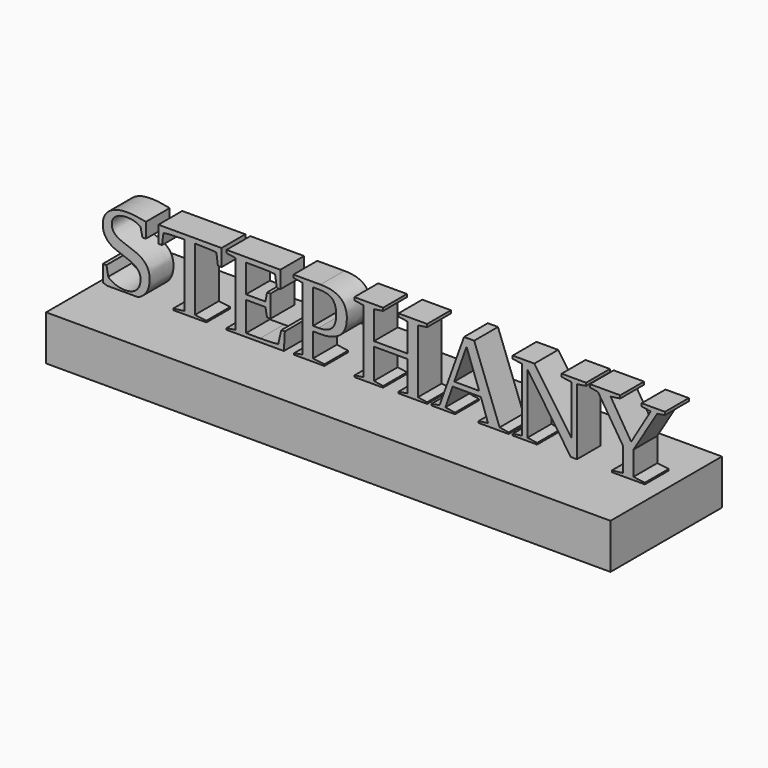
from build123d import *

# Parameters (mm, degrees)
F0_TEXT_SIZE  = 46.7684339835
F1_DEPTH      = 12.7
F2_W          = 240.8891022205
F2_H          = 19.2134454846
F3_DEPTH      = 40.386
F3_DEPTH_BACK = 19.05


# Not quite as in the source:
# - Text() gives the source's letters only with a copy of the font that has no kerning and outlines rounded to 1/6400 em; it was checked with that copy


with BuildPart() as f1:
    # F0 (on Front) → F1 (new body)
    with BuildSketch(Plane.XZ):
        with Locations((-124.9077068642, -14.3902879208)):
            Text('STEPHANY', F0_TEXT_SIZE, font='Tinos', text_align=(TextAlign.LEFT, TextAlign.BOTTOM))
    extrude(amount=F1_DEPTH)


with BuildPart() as f3:
    # F2 (on Front) → F3 (new body, two sides)
    with BuildSketch(Plane.XZ) as f3_sk:
        with Locations((-3.39615345, -23.4213992953)):
            Rectangle(F2_W, F2_H)
    extrude(amount=F3_DEPTH)
    extrude(f3_sk.sketch, amount=-F3_DEPTH_BACK)


solid = Compound([f1.part, f3.part])
